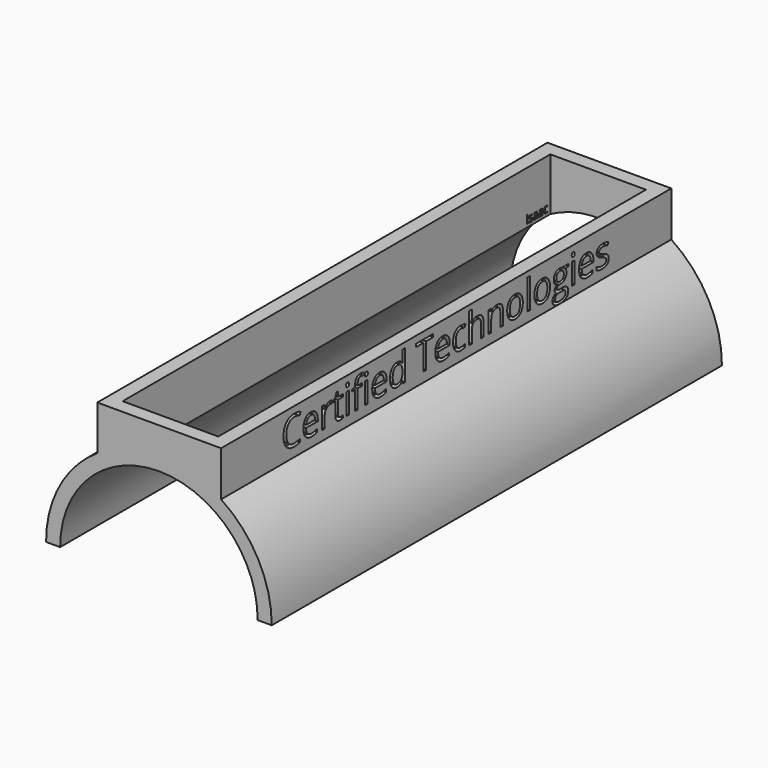
from build123d import *

# Parameters (mm, degrees)
F1_DEPTH     = 254
F2_W         = 43.18
F2_H         = 241.3
F3_DEPTH     = 25.4
F4_TEXT_SIZE = 17.9147192587
F5_DEPTH     = 2.54
F6_TEXT_SIZE = 5.2916666667
F7_DEPTH     = 2.54


# Not quite as in the source:
# - Text() gives the source's letters only with a copy of the font that has no kerning and outlines rounded to 1/6400 em; it was checked with that copy


with BuildPart() as f1:
    # F0 (on Front) → F1 (new body)
    with BuildSketch(Plane.XZ):
        with BuildLine():
            ThreePointArc((-44.7086496091, 0), (-0.1316496091, 44.6969019903), (44.4453503909, 0))
            Line((44.4453503909, 0), (50.7953274818, -0.0170570849))
            ThreePointArc((50.7953274818, -0.0170570849), (44.7514918708, 24.1838081621), (27.94, 42.6116015372))
            Line((27.94, 42.6116015372), (27.94, 62.9316015372))
            Line((27.94, 62.9316015372), (21.59, 62.9316015372))
            Line((21.59, 62.9316015372), (-21.59, 62.9316015372))
            Line((-21.59, 62.9316015372), (-27.94, 62.9316015372))
            Line((-27.94, 62.9316015372), (-27.94, 42.7843794291))
            ThreePointArc((-27.94, 42.7843794291), (-44.9401721281, 24.322468681), (-51.0586267001, -0.0170570849))
            Line((-51.0586267001, -0.0170570849), (-44.7086496091, 0))
        make_face()
    extrude(amount=-F1_DEPTH)

    # F2 (on face) → F3 (cut)
    with BuildSketch(Plane.XY.offset(62.9316015372)):
        with Locations((0, 127)):
            Rectangle(F2_W, F2_H)
    extrude(amount=-F3_DEPTH, mode=Mode.SUBTRACT)

    # F4 (on face) → F5 (cut)
    with BuildSketch(Plane.YZ.offset(27.94)):
        with Locations((34.1233773429, 46.9507947564)):
            Text('Certified Technologies', F4_TEXT_SIZE, font='Open Sans', text_align=(TextAlign.LEFT, TextAlign.BOTTOM))
    extrude(amount=-F5_DEPTH, mode=Mode.SUBTRACT)

    # F6 (on face) → F7 (cut)
    with BuildSketch(Plane.YZ.offset(-21.59)):
        with Locations((233.9043538146, 40.5044555556)):
            Text('Isaac', F6_TEXT_SIZE, font='Open Sans', text_align=(TextAlign.LEFT, TextAlign.BOTTOM))
    extrude(amount=-F7_DEPTH, mode=Mode.SUBTRACT)


solid = f1.part
